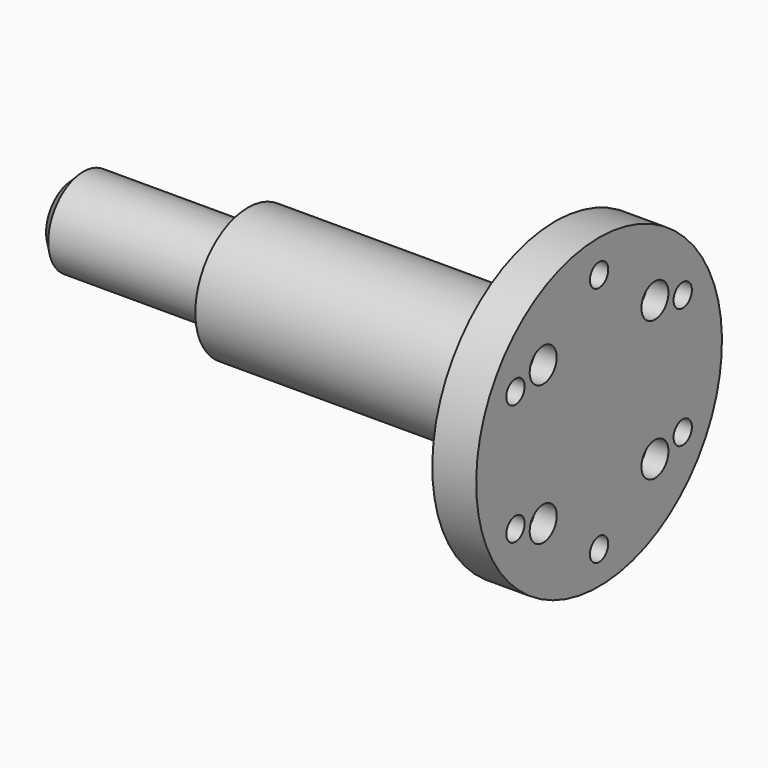
from build123d import *

# Parameters (mm, degrees)
F2_R             = 3.175
F3_R             = 3.175
F4_SIZE          = 3.175
F5_R             = 3.3147
F6_DEPTH         = 152.401
F6_COPIES_COUNT  = 6
F7_W             = 3.175
F7_H             = 3.175
F8_DEPTH         = 25.4
F9_R             = 4.8895
F10_DEPTH        = 152.401
F10_COPIES_COUNT = 4
F11_R            = 6.35
F12_DEPTH        = 6.35
F12_COPIES_COUNT = 4


# Not quite as in the source:
# - a pattern or mirror of a feature is missing from the dataset's text; its kind, count and spacing are read off the source's solid


with BuildPart() as f1:
    # F0 (on Front) → F1 (revolve)
    with BuildSketch(Plane.XZ):
        Polygon((0, 12.7), (0, 0), (152.4, 0), (152.4, 44.45), (139.7, 44.45), (139.7, 19.05), (50.8, 19.05), (50.8, 12.7), align=None)
    revolve(axis=Axis((76.2, 0, 0), (1, 0, 0)))

    # F2
    f2_edges = [f1.edges().sort_by_distance(p)[0] for p in [
        (50.8, 0, -12.7),
    ]]
    fillet(f2_edges, radius=F2_R)

    # F3
    f3_edges = [f1.edges().sort_by_distance(p)[0] for p in [
        (139.7, 0, -19.05),
    ]]
    fillet(f3_edges, radius=F3_R)

    # F4
    f4_edges = [f1.edges().sort_by_distance(p)[0] for p in [
        (0, 0, -12.7),
    ]]
    chamfer(f4_edges, length=F4_SIZE)

    # F5 (on face) → F6 (cut, through all)
    with BuildSketch(Plane.YZ.offset(152.4)):
        with Locations((0, -34.925)):
            Circle(F5_R)
    f6 = extrude(amount=-F6_DEPTH, mode=Mode.SUBTRACT)

    # F6_copies: F6 ×6 about axis
    f6_copies_axis = Axis((0, 0, 0), (1, 0, 0))
    for i in range(1, F6_COPIES_COUNT):
        add(f6.rotate(f6_copies_axis, i * 360 / F6_COPIES_COUNT), mode=Mode.SUBTRACT)

    # F7 (on face) → F8 (cut)
    with BuildSketch(Plane(origin=(50.8, 0, 0), x_dir=(0, -1, 0), z_dir=(-1, 0, 0))):
        with Locations((1.5875, -17.4625)):
            Rectangle(F7_W, F7_H)
        with Locations((-1.5875, -17.4625)):
            Rectangle(F7_W, F7_H)
    extrude(amount=-F8_DEPTH, mode=Mode.SUBTRACT)

    # F9 (on face) → F10 (cut, through all)
    with BuildSketch(Plane.YZ.offset(152.4)):
        with Locations((-20.2055762724, -20.2055762724)):
            Circle(F9_R)
    f10 = extrude(amount=-F10_DEPTH, mode=Mode.SUBTRACT)

    # F10_copies: F10 ×4 about axis
    f10_copies_axis = Axis((0, 0, 0), (1, 0, 0))
    for i in range(1, F10_COPIES_COUNT):
        add(f10.rotate(f10_copies_axis, i * 360 / F10_COPIES_COUNT), mode=Mode.SUBTRACT)

    # F11 (on face) → F12 (cut)
    with BuildSketch(Plane(origin=(139.7, 0, 0), x_dir=(0, -1, 0), z_dir=(-1, 0, 0))):
        with Locations((20.2055762724, -20.2055762724)):
            Circle(F11_R)
    f12 = extrude(amount=-F12_DEPTH, mode=Mode.SUBTRACT)

    # F12_copies: F12 ×4 about axis
    f12_copies_axis = Axis((0, 0, 0), (1, 0, 0))
    for i in range(1, F12_COPIES_COUNT):
        add(f12.rotate(f12_copies_axis, i * 360 / F12_COPIES_COUNT), mode=Mode.SUBTRACT)


solid = f1.part
